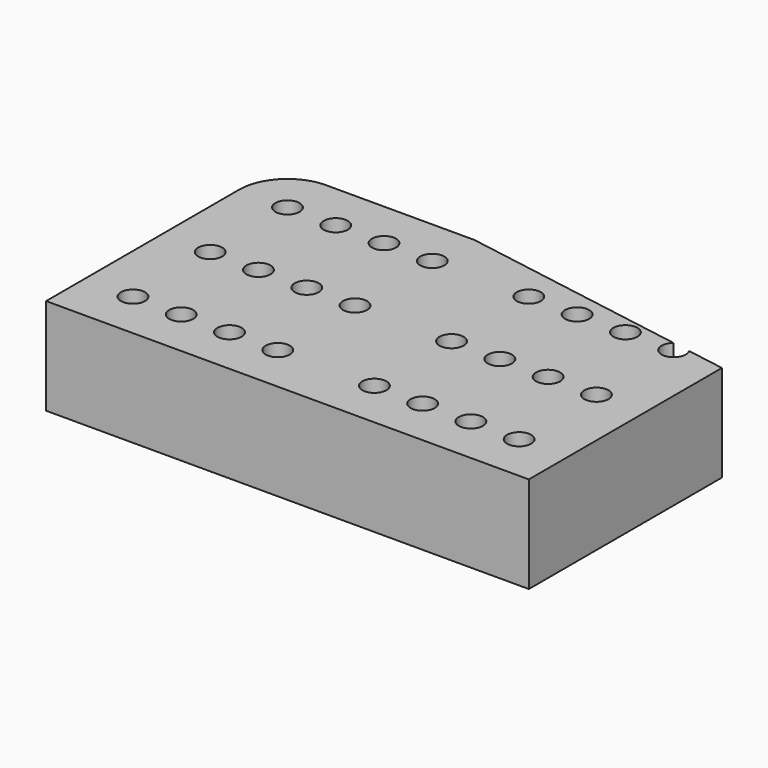
from build123d import *

# Parameters (mm, degrees)
F1_DEPTH = 25.4
F2_R     = 3.175
F3_DEPTH = 25.4
F4_T     = -2.54


# Not quite as in the source:
# - a shell that OpenCascade refuses in one call is made with other operations: the cavity is built on its own and cut out


with BuildPart() as f1:
    # F0 (on Top) → F1 (new body)
    with BuildSketch(Plane.XY):
        with BuildLine():
            Line((51.71799147, 0), (12.7, 0))
            ThreePointArc((12.7, 0), (3.7197438789, -3.7197438789), (0, -12.7))
            Line((0, -12.7), (0, -76.2))
            Line((0, -76.2), (127, -76.2))
            Line((127, -76.2), (127, -12.7))
            Line((127, -12.7), (51.71799147, 0))
        make_face()
    extrude(amount=F1_DEPTH)

    # F2 (on face) → F3 (cut)
    with BuildSketch(Plane.XY.offset(25.4)):
        with Locations((12.7, -12.7)):
            Circle(F2_R)
        with Locations((12.7, -38.1)):
            Circle(F2_R)
        with Locations((12.7, -63.5)):
            Circle(F2_R)
        with Locations((25.4, -12.7)):
            Circle(F2_R)
        with Locations((25.4, -38.1)):
            Circle(F2_R)
        with Locations((25.4, -63.5)):
            Circle(F2_R)
        with Locations((38.1, -12.7)):
            Circle(F2_R)
        with Locations((38.1, -38.1)):
            Circle(F2_R)
        with Locations((38.1, -63.5)):
            Circle(F2_R)
        with Locations((50.8, -12.7)):
            Circle(F2_R)
        with Locations((50.8, -38.1)):
            Circle(F2_R)
        with Locations((50.8, -63.5)):
            Circle(F2_R)
        with Locations((114.3, -12.7)):
            Circle(F2_R)
        with Locations((101.6, -12.7)):
            Circle(F2_R)
        with Locations((88.9, -12.7)):
            Circle(F2_R)
        with Locations((114.3, -38.1)):
            Circle(F2_R)
        with Locations((101.6, -38.1)):
            Circle(F2_R)
        with Locations((88.9, -38.1)):
            Circle(F2_R)
        with Locations((114.3, -63.5)):
            Circle(F2_R)
        with Locations((101.6, -63.5)):
            Circle(F2_R)
        with Locations((88.9, -63.5)):
            Circle(F2_R)
        with Locations((76.2, -63.5)):
            Circle(F2_R)
        with Locations((76.2, -38.1)):
            Circle(F2_R)
        with Locations((76.2, -12.7)):
            Circle(F2_R)
    extrude(amount=-F3_DEPTH, mode=Mode.SUBTRACT)

    # F4: a shell. OpenCascade refuses it in one call, so the cavity is built on its own and cut out:
    # the body offset inwards by the wall thickness, plus a prism from it out through each open face.
    f4_core = offset(f1.part, amount=F4_T, kind=Kind.INTERSECTION, mode=Mode.PRIVATE)
    f4_exits = [f4_core.faces().sort_by_distance(p)[0] for p in [
        (61.661975, -40.163324, 2.54),
    ]]
    add(f4_core, mode=Mode.SUBTRACT)
    extrude(f4_exits, amount=-F4_T, mode=Mode.SUBTRACT)


solid = f1.part
